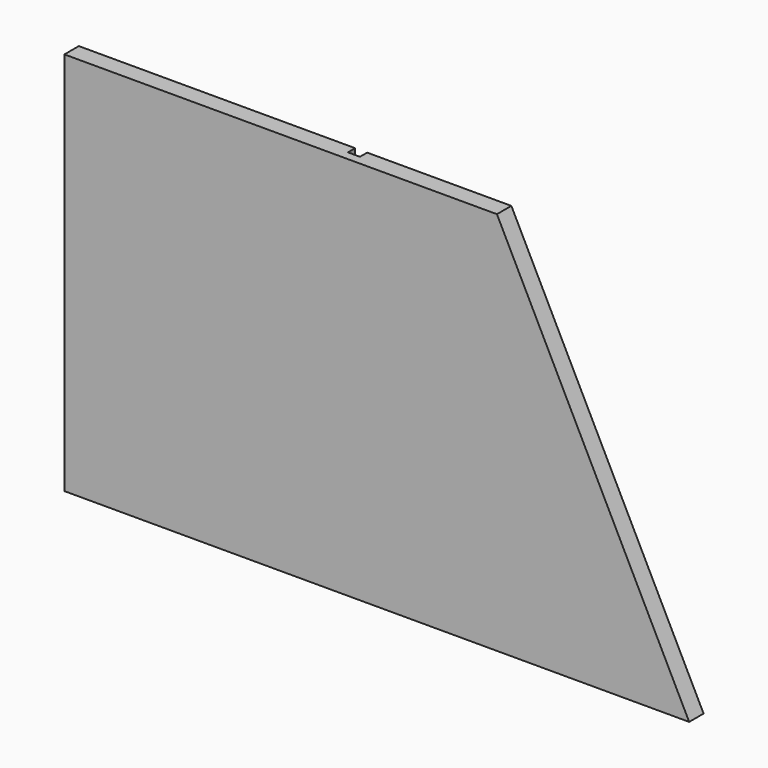
from build123d import *

# Parameters (mm, degrees)
F1_DEPTH = 19.05
F2_W     = 12.7
F2_H     = 406.4
F3_DEPTH = 9.525


# Not quite as in the source:
# - a feature names something its author has since deleted; it is built from what else it names


with BuildPart() as f1:
    # F0 (on Front) → F1 (new body)
    with BuildSketch(Plane.XZ):
        Polygon((-229.6549332498, 252.4134865394), (-356.6549332498, 252.4134865394), (-686.8549332498, 252.4134865394), (-686.8549332498, -153.9865134606), (-356.6549332498, -153.9865134606), (-26.4549332498, -153.9865134606), align=None)
    extrude(amount=F1_DEPTH)

    # F2 (on face) → F3 (cut)
    with BuildSketch(Plane(origin=(0, 0, 0), x_dir=(-1, 0, 0), z_dir=(0, 1, 0))):
        with Locations((388.4049332498, 49.2134865394)):
            Rectangle(F2_W, F2_H)
    extrude(amount=-F3_DEPTH, mode=Mode.SUBTRACT)


solid = f1.part
